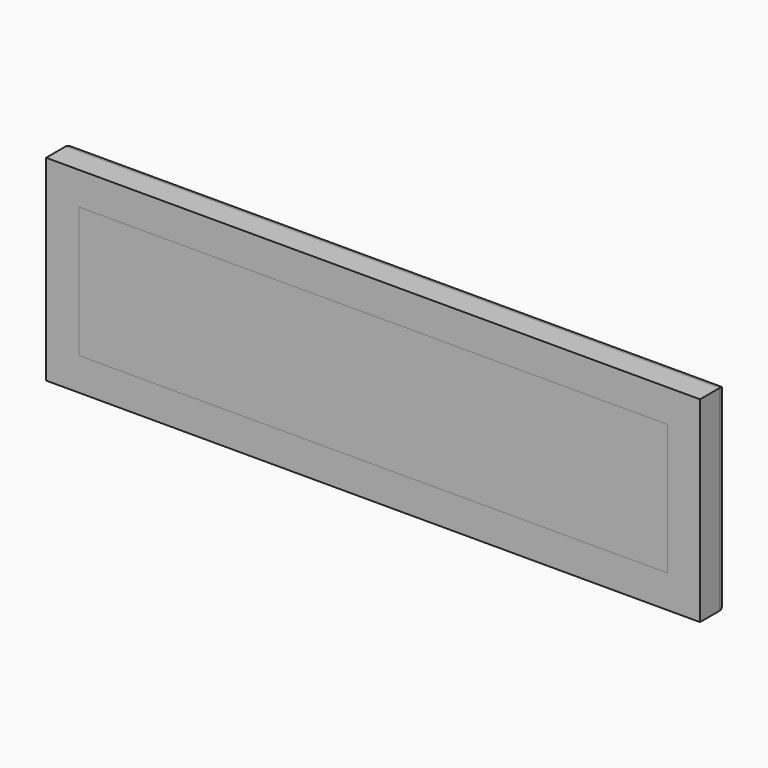
from build123d import *

# Parameters (mm, degrees)
F0_W         = 100
F0_H         = 30
F0_W_2       = 90
F0_H_2       = 20
F1_DEPTH     = 5
F2_DEPTH     = 2.5
F3_R         = 1.25
F4_TEXT_SIZE = 18.2199921711
F5_DEPTH     = 2.5


# Not quite as in the source:
# - Text() gives the source's letters only with a copy of the font that has no kerning and outlines rounded to 1/6400 em; it was checked with that copy


with BuildPart() as f1:
    # F0 (on Front) → F1 (new body)
    with BuildSketch(Plane.XZ):
        Rectangle(F0_W, F0_H)
        Rectangle(F0_W_2, F0_H_2, mode=Mode.SUBTRACT)
    extrude(amount=-F1_DEPTH)

    # F3
    f3_edges = [f1.edges().sort_by_distance(p)[0] for p in [
        (0, 5, 15),
        (50, 5, 0),
        (0, 5, -15),
        (-50, 5, 0),
    ]]
    fillet(f3_edges, radius=F3_R)


with BuildPart() as f2:
    # F0 (on Front) → F2 (new body)
    with BuildSketch(Plane.XZ):
        Rectangle(F0_W_2, F0_H_2)
    extrude(amount=-F2_DEPTH)

    # F4 (on face) → F5 (join)
    with BuildSketch(Plane(origin=(0, 2.5, 0), x_dir=(-1, 0, 0), z_dir=(0, 1, 0))):
        with Locations((-38.4830832481, -4.4403420761)):
            Text('Mr. Haney', F4_TEXT_SIZE, font='Tinos', text_align=(TextAlign.LEFT, TextAlign.BOTTOM))
    extrude(amount=F5_DEPTH)


solid = Compound([f1.part, f2.part])
